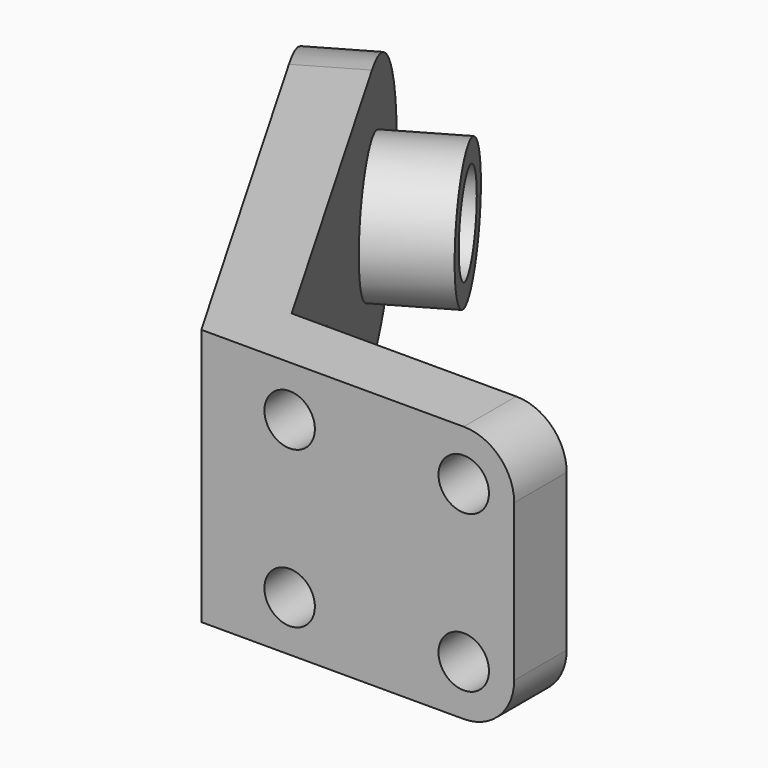
from build123d import *

# Parameters (mm, degrees)
F1_DEPTH  = 102
F2_R      = 50.99999
F3_R      = 27
F3_R_2    = 18.5
F4_DEPTH  = 30
F8_DEPTH  = 10
F5_R      = 10
F9_DEPTH  = 30
F10_R     = 18.5
F11_DEPTH = 30
F12_R     = 20
F13_R     = 20


# Not quite as in the source:
# - a fillet or chamfer is up to 0.001 mm smaller than in the source, because OpenCascade refuses the exact size


with BuildPart() as f1:
    # F0 (on Top) → F1 (new body)
    with BuildSketch(Plane.XY):
        Polygon((-3.5224159509, -94.9145984159), (-111.5168624514, 92.1372698583), (-134.0335229498, 79.1372698583), (-18.5335229498, -120.9145984159), (105.4775840491, -120.9145984159), (105.4775840491, -94.9145984159), align=None)
    extrude(amount=F1_DEPTH)

    # F2 (radius 51 in the source; OpenCascade refuses exactly that, so slightly less here)
    f2_edges = [f1.edges().sort_by_distance(p)[0] for p in [
        (-122.775193, 85.63727, 102),
        (-122.775193, 85.63727, 0),
    ]]
    fillet(f2_edges, radius=F2_R)

    # F3 (on face) → F4 (join)
    with BuildSketch(Plane(origin=(-43.7410386722, -25.253900452, 0), x_dir=(-0.5, 0.8660254038, 0), z_dir=(0.8660254038, 0.5, 0))):
        with Locations((84.5516475584, 51)):
            Circle(F3_R)
        with Locations((84.5516475584, 51)):
            Circle(F3_R_2, mode=Mode.SUBTRACT)
    extrude(amount=F4_DEPTH)

    # F7 (on offset) → F8 (join, symmetric)
    with BuildSketch(Plane.XY.offset(51)):
        Polygon((-3.5224159509, -94.9145984159), (105.4775840491, -94.9145984159), (-44.2564783831, -30.7528017003), align=None)
    extrude(amount=F8_DEPTH, both=True)

    # F5 (on face) → F9 (cut)
    with BuildSketch(Plane(origin=(0, -94.9145984159, 0), x_dir=(-1, 0, 0), z_dir=(0, 1, 0))):
        with Locations((-85.4775840491, 82)):
            Circle(F5_R)
        with Locations((-85.4775840491, 20)):
            Circle(F5_R)
        with Locations((-16.4775840491, 82)):
            Circle(F5_R)
        with Locations((-16.4775840491, 20)):
            Circle(F5_R)
    extrude(amount=-F9_DEPTH, mode=Mode.SUBTRACT)

    # F10 (on face) → F11 (cut)
    with BuildSketch(Plane(origin=(-43.7410386722, -25.253900452, 0), x_dir=(-0.5, 0.8660254038, 0), z_dir=(0.8660254038, 0.5, 0))):
        with Locations((84.5516475584, 51)):
            Circle(F10_R)
    extrude(amount=-F11_DEPTH, mode=Mode.SUBTRACT)

    # F12
    f12_edges = [f1.edges().sort_by_distance(p)[0] for p in [
        (105.477584, -107.914598, 102),
    ]]
    fillet(f12_edges, radius=F12_R)

    # F13
    f13_edges = [f1.edges().sort_by_distance(p)[0] for p in [
        (105.477584, -107.914598, 0),
    ]]
    fillet(f13_edges, radius=F13_R)


solid = f1.part
